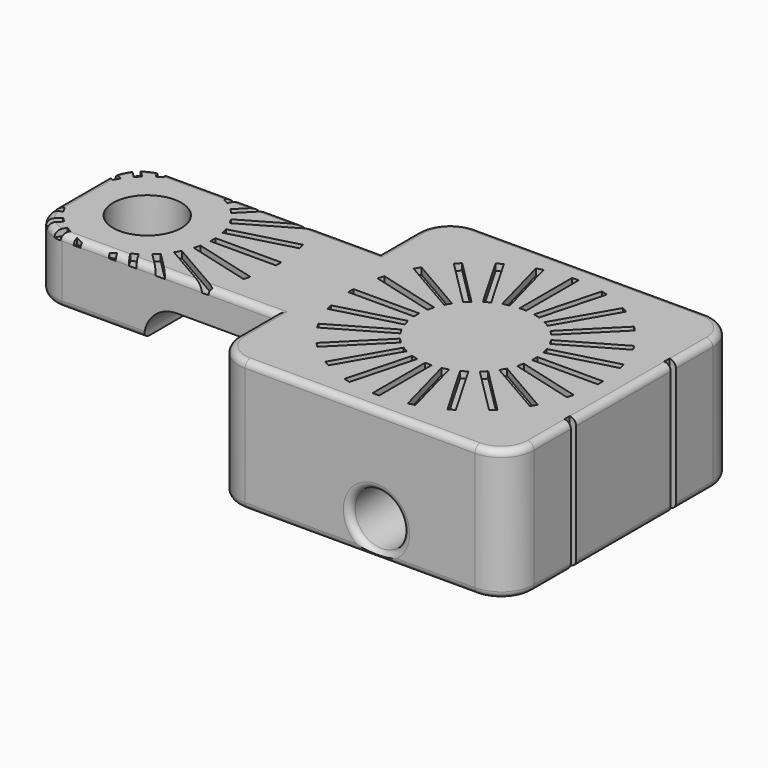
from build123d import *

# Parameters (mm, degrees)
F0_R         = 5.2
F1_DEPTH     = 20
F2_W         = 37.5
F2_H         = 20
F3_DEPTH     = 10
F4_R         = 4.05
F5_DEPTH     = 10
F6_R         = 4.05
F7_DEPTH     = 10
F8_T1_DEPTH  = 35
F8_T3_DEPTH  = 34
F8_T5_DEPTH  = 10
F8_T7_DEPTH  = 32.5
F8_T9_DEPTH  = 7
F8_T11_DEPTH = 7
F8_T14_ANGLE = 90
F8_T16_ANGLE = 90
F8_T18_ANGLE = 90
F8_T20_ANGLE = 90
F8_T26_ANGLE = 90
F8_T28_ANGLE = 90
F8_T30_ANGLE = 90
F8_T32_ANGLE = 90
F8_T34_ANGLE = 90
F8_T36_ANGLE = 90
F8_T38_ANGLE = 90
F8_T40_ANGLE = 90
F8_T45_DEPTH = 35
F8_T49_DEPTH = 9.5
F8_T56_DEPTH = 9.5
F8_T60_DEPTH = 35
F10_DEPTH    = 1
F11_W        = 20
F11_H        = 5
F12_DEPTH    = 32.0010001
F13_R        = 4.99999
F14_W        = 10
F14_H        = 1
F14_W_2      = 1
F14_H_2      = 10
F15_DEPTH    = 1
F16_W        = 2
F16_H        = 1
F17_DEPTH    = 20.0010001


# Not quite as in the source:
# - a fillet or chamfer that OpenCascade refuses, or shapes differently, is made with other operations: its cross-section is extruded or revolved along the edge and cut away or added
# - a fillet or chamfer is up to 0.001 mm smaller than in the source, because OpenCascade refuses the exact size


with BuildPart() as f1:
    # F0 (on Top) → F1 (new body)
    with BuildSketch(Plane.XY):
        with BuildLine():
            Line((-17.5, -22), (17.5, -22))
            ThreePointArc((17.5, -22), (21.0355339059, -20.5355339059), (22.5, -17))
            Line((22.5, -17), (22.5, 17))
            ThreePointArc((22.5, 17), (21.0355339059, 20.5355339059), (17.5, 22))
            Line((17.5, 22), (-17.5, 22))
            ThreePointArc((-17.5, 22), (-21.0355339059, 20.5355339059), (-22.5, 17))
            Line((-22.5, 17), (-22.5, 10))
            Line((-22.5, 10), (-55, 10))
            ThreePointArc((-55, 10), (-58.5355339059, 8.5355339059), (-60, 5))
            Line((-60, 5), (-60, -5))
            ThreePointArc((-60, -5), (-58.5355339059, -8.5355339059), (-55, -10))
            Line((-55, -10), (-22.5, -10))
            Line((-22.5, -10), (-22.5, -17))
            ThreePointArc((-22.5, -17), (-21.0355339059, -20.5355339059), (-17.5, -22))
        make_face()
        with Locations((-50, 0)):
            Circle(F0_R, mode=Mode.SUBTRACT)
    extrude(amount=F1_DEPTH)

    # F2 (on face) → F3 (cut)
    with BuildSketch(Plane(origin=(0, 0, 0), x_dir=(1, 0, 0), z_dir=(0, 0, -1))):
        with Locations((-41.25, 0)):
            Rectangle(F2_W, F2_H)
    extrude(amount=-F3_DEPTH, mode=Mode.SUBTRACT)

    # F4 (on face) → F5 (cut)
    with BuildSketch(Plane.XZ.offset(22)):
        with Locations((2.5, 5)):
            Circle(F4_R)
    extrude(amount=-F5_DEPTH, mode=Mode.SUBTRACT)

    # F6 (on face) → F7 (cut)
    with BuildSketch(Plane(origin=(0, 22, 0), x_dir=(-1, 0, 0), z_dir=(0, 1, 0))):
        with Locations((-2.5, 5)):
            Circle(F6_R)
    extrude(amount=-F7_DEPTH, mode=Mode.SUBTRACT)

    # F8: fillet of radius 1 on 18 edges, made by hand

    # F8_s2 → F8_t1 (cut)
    with BuildSketch(Plane.YZ.offset(-17.5)):
        with BuildLine():
            ThreePointArc((-22, 1), (-21.7071067812, 0.2928932188), (-21, 0))
            Line((-21, 0), (-22, 0))
            Line((-22, 0), (-22, 1))
        make_face()
        with BuildLine():
            ThreePointArc((21, 0), (21.7071067812, 0.2928932188), (22, 1))
            Line((22, 1), (22, 0))
            Line((22, 0), (21, 0))
        make_face()
        with BuildLine():
            ThreePointArc((21, 20), (21.7071067812, 19.7071067812), (22, 19))
            Line((22, 19), (22, 20))
            Line((22, 20), (21, 20))
        make_face()
        with BuildLine():
            ThreePointArc((-22, 19), (-21.7071067812, 19.7071067812), (-21, 20))
            Line((-21, 20), (-22, 20))
            Line((-22, 20), (-22, 19))
        make_face()
    extrude(amount=F8_T1_DEPTH, mode=Mode.SUBTRACT)

    # F8_s4 → F8_t3 (cut)
    with BuildSketch(Plane.XZ.offset(-17)):
        with BuildLine():
            ThreePointArc((21.5, 0), (22.2071067812, 0.2928932188), (22.5, 1))
            Line((22.5, 1), (22.5, 0))
            Line((22.5, 0), (21.5, 0))
        make_face()
        with BuildLine():
            ThreePointArc((-21.5, 0), (-22.2071067812, 0.2928932188), (-22.5, 1))
            Line((-22.5, 1), (-22.5, 0))
            Line((-22.5, 0), (-21.5, 0))
        make_face()
        with BuildLine():
            ThreePointArc((21.5, 20), (22.2071067812, 19.7071067812), (22.5, 19))
            Line((22.5, 19), (22.5, 20))
            Line((22.5, 20), (21.5, 20))
        make_face()
    extrude(amount=F8_T3_DEPTH, mode=Mode.SUBTRACT)

    # F8_s6 → F8_t5 (cut)
    with BuildSketch(Plane.XZ.offset(-5)):
        with BuildLine():
            ThreePointArc((-60, 11), (-59.7071067812, 10.2928932188), (-59, 10))
            Line((-59, 10), (-60, 10))
            Line((-60, 10), (-60, 11))
        make_face()
        with BuildLine():
            ThreePointArc((-59, 20), (-59.7071067812, 19.7071067812), (-60, 19))
            Line((-60, 19), (-60, 20))
            Line((-60, 20), (-59, 20))
        make_face()
    extrude(amount=F8_T5_DEPTH, mode=Mode.SUBTRACT)

    # F8_s8 → F8_t7 (cut)
    with BuildSketch(Plane.YZ.offset(-55)):
        with BuildLine():
            ThreePointArc((-9, 20), (-9.7071067812, 19.7071067812), (-10, 19))
            Line((-10, 19), (-10, 20))
            Line((-10, 20), (-9, 20))
        make_face()
        with BuildLine():
            ThreePointArc((9, 20), (9.7071067812, 19.7071067812), (10, 19))
            Line((10, 19), (10, 20))
            Line((10, 20), (9, 20))
        make_face()
        with BuildLine():
            ThreePointArc((10, 11), (9.7071067812, 10.2928932188), (9, 10))
            Line((9, 10), (10, 10))
            Line((10, 10), (10, 11))
        make_face()
        with BuildLine():
            ThreePointArc((-10, 11), (-9.7071067812, 10.2928932188), (-9, 10))
            Line((-9, 10), (-10, 10))
            Line((-10, 10), (-10, 11))
        make_face()
    extrude(amount=F8_T7_DEPTH, mode=Mode.SUBTRACT)

    # F8_s10 → F8_t9 (cut)
    with BuildSketch(Plane.XZ.offset(10)):
        with BuildLine():
            ThreePointArc((-21.5, 20), (-22.2071067812, 19.7071067812), (-22.5, 19))
            Line((-22.5, 19), (-22.5, 20))
            Line((-22.5, 20), (-21.5, 20))
        make_face()
    extrude(amount=F8_T9_DEPTH, mode=Mode.SUBTRACT)

    # F8_s12 → F8_t11 (cut)
    with BuildSketch(Plane.XZ.offset(-17)):
        with BuildLine():
            ThreePointArc((-21.5, 20), (-22.2071067812, 19.7071067812), (-22.5, 19))
            Line((-22.5, 19), (-22.5, 20))
            Line((-22.5, 20), (-21.5, 20))
        make_face()
    extrude(amount=F8_T11_DEPTH, mode=Mode.SUBTRACT)

    # F8_s13 → F8_t14 (revolve, cut)
    with BuildSketch(Plane.XZ.offset(17)):
        with BuildLine():
            ThreePointArc((-22.5, 1), (-22.2071067812, 0.2928932188), (-21.5, 0))
            Line((-21.5, 0), (-22.5, 0))
            Line((-22.5, 0), (-22.5, 1))
        make_face()
    revolve(axis=Axis((-17.5, -17, 0), (0, 0, 1)), revolution_arc=F8_T14_ANGLE, mode=Mode.SUBTRACT)

    # F8_s15 → F8_t16 (revolve, cut)
    with BuildSketch(Plane.YZ.offset(17.5)):
        with BuildLine():
            ThreePointArc((-21, 0), (-21.7071067812, 0.2928932188), (-22, 1))
            Line((-22, 1), (-22, 0))
            Line((-22, 0), (-21, 0))
        make_face()
    revolve(axis=Axis((17.5, -17, 0), (0, 0, 1)), revolution_arc=F8_T16_ANGLE, mode=Mode.SUBTRACT)

    # F8_s17 → F8_t18 (revolve, cut)
    with BuildSketch(Plane.XZ.offset(-17)):
        with BuildLine():
            ThreePointArc((21.5, 0), (22.2071067812, 0.2928932188), (22.5, 1))
            Line((22.5, 1), (22.5, 0))
            Line((22.5, 0), (21.5, 0))
        make_face()
    revolve(axis=Axis((17.5, 17, 0), (0, 0, 1)), revolution_arc=F8_T18_ANGLE, mode=Mode.SUBTRACT)

    # F8_s19 → F8_t20 (revolve, cut)
    with BuildSketch(Plane.YZ.offset(-17.5)):
        with BuildLine():
            ThreePointArc((21, 0), (21.7071067812, 0.2928932188), (22, 1))
            Line((22, 1), (22, 0))
            Line((22, 0), (21, 0))
        make_face()
    revolve(axis=Axis((-17.5, 17, 0), (0, 0, 1)), revolution_arc=F8_T20_ANGLE, mode=Mode.SUBTRACT)

    # F8_s21 → F8_t22 (revolve, cut)
    with BuildSketch(Plane.XY.offset(5)):
        with BuildLine():
            ThreePointArc((7.55, -22), (6.8428932188, -21.7071067812), (6.55, -21))
            Line((6.55, -21), (6.55, -22))
            Line((6.55, -22), (7.55, -22))
        make_face()
    revolve(axis=Axis((2.5, -22, 5), (0, -1, 0)), mode=Mode.SUBTRACT)

    # F8_s23 → F8_t24 (revolve, cut)
    with BuildSketch(Plane.XY.offset(5)):
        with BuildLine():
            ThreePointArc((-2.55, 22), (-1.8428932188, 21.7071067812), (-1.55, 21))
            Line((-1.55, 21), (-1.55, 22))
            Line((-1.55, 22), (-2.55, 22))
        make_face()
    revolve(axis=Axis((2.5, 22, 5), (0, 1, 0)), mode=Mode.SUBTRACT)

    # F8_s25 → F8_t26 (revolve, cut)
    with BuildSketch(Plane.XZ.offset(17)):
        with BuildLine():
            ThreePointArc((-22.5, 19), (-22.2071067812, 19.7071067812), (-21.5, 20))
            Line((-21.5, 20), (-22.5, 20))
            Line((-22.5, 20), (-22.5, 19))
        make_face()
    revolve(axis=Axis((-17.5, -17, 20), (0, 0, 1)), revolution_arc=F8_T26_ANGLE, mode=Mode.SUBTRACT)

    # F8_s27 → F8_t28 (revolve, cut)
    with BuildSketch(Plane.YZ.offset(17.5)):
        with BuildLine():
            ThreePointArc((-21, 20), (-21.7071067812, 19.7071067812), (-22, 19))
            Line((-22, 19), (-22, 20))
            Line((-22, 20), (-21, 20))
        make_face()
    revolve(axis=Axis((17.5, -17, 20), (0, 0, 1)), revolution_arc=F8_T28_ANGLE, mode=Mode.SUBTRACT)

    # F8_s29 → F8_t30 (revolve, cut)
    with BuildSketch(Plane.XZ.offset(-17)):
        with BuildLine():
            ThreePointArc((21.5, 20), (22.2071067812, 19.7071067812), (22.5, 19))
            Line((22.5, 19), (22.5, 20))
            Line((22.5, 20), (21.5, 20))
        make_face()
    revolve(axis=Axis((17.5, 17, 20), (0, 0, 1)), revolution_arc=F8_T30_ANGLE, mode=Mode.SUBTRACT)

    # F8_s31 → F8_t32 (revolve, cut)
    with BuildSketch(Plane.YZ.offset(-17.5)):
        with BuildLine():
            ThreePointArc((21, 20), (21.7071067812, 19.7071067812), (22, 19))
            Line((22, 19), (22, 20))
            Line((22, 20), (21, 20))
        make_face()
    revolve(axis=Axis((-17.5, 17, 20), (0, 0, 1)), revolution_arc=F8_T32_ANGLE, mode=Mode.SUBTRACT)

    # F8_s33 → F8_t34 (revolve, cut)
    with BuildSketch(Plane.XZ.offset(5)):
        with BuildLine():
            ThreePointArc((-59, 20), (-59.7071067812, 19.7071067812), (-60, 19))
            Line((-60, 19), (-60, 20))
            Line((-60, 20), (-59, 20))
        make_face()
    revolve(axis=Axis((-55, -5, 20), (0, 0, 1)), revolution_arc=F8_T34_ANGLE, mode=Mode.SUBTRACT)

    # F8_s35 → F8_t36 (revolve, cut)
    with BuildSketch(Plane.YZ.offset(-55)):
        with BuildLine():
            ThreePointArc((9, 20), (9.7071067812, 19.7071067812), (10, 19))
            Line((10, 19), (10, 20))
            Line((10, 20), (9, 20))
        make_face()
    revolve(axis=Axis((-55, 5, 20), (0, 0, 1)), revolution_arc=F8_T36_ANGLE, mode=Mode.SUBTRACT)

    # F8_s37 → F8_t38 (revolve, cut)
    with BuildSketch(Plane.YZ.offset(-55)):
        with BuildLine():
            ThreePointArc((-10, 11), (-9.7071067812, 10.2928932188), (-9, 10))
            Line((-9, 10), (-10, 10))
            Line((-10, 10), (-10, 11))
        make_face()
    revolve(axis=Axis((-55, -5, 10), (0, 0, -1)), revolution_arc=F8_T38_ANGLE, mode=Mode.SUBTRACT)

    # F8_s39 → F8_t40 (revolve, cut)
    with BuildSketch(Plane.XZ.offset(-5)):
        with BuildLine():
            ThreePointArc((-60, 11), (-59.7071067812, 10.2928932188), (-59, 10))
            Line((-59, 10), (-60, 10))
            Line((-60, 10), (-60, 11))
        make_face()
    revolve(axis=Axis((-55, 5, 10), (0, 0, -1)), revolution_arc=F8_T40_ANGLE, mode=Mode.SUBTRACT)


with BuildPart() as f8_tool43:
    # F8_s44 → F8_t45 (new body)
    with BuildSketch(Plane.YZ.offset(-55)):
        with BuildLine():
            ThreePointArc((-9, 20), (-9.7071067812, 19.7071067812), (-10, 19))
            Line((-10, 19), (-10, 20))
            Line((-10, 20), (-9, 20))
        make_face()
    extrude(amount=F8_T45_DEPTH)

    split(bisect_by=Plane.YZ.offset(-22.5), keep=Keep.TOP)


with BuildPart() as f8_tool47:
    # F8_s48 → F8_t49 (new body)
    with BuildSketch(Plane.XZ.offset(7.5)):
        with BuildLine():
            ThreePointArc((-21.5, 20), (-22.2071067812, 19.7071067812), (-22.5, 19))
            Line((-22.5, 19), (-22.5, 20))
            Line((-22.5, 20), (-21.5, 20))
        make_face()
    extrude(amount=F8_T49_DEPTH)

    split(bisect_by=Plane.XZ.offset(10), keep=Keep.BOTTOM)


with BuildPart() as f8_tool43_1:
    add(f8_tool43.part)

    # F8_t51: intersect F8_tool47
    add(f8_tool47.part, mode=Mode.INTERSECT)


with BuildPart() as f1_1:
    add(f1.part)

    # F8_t41: cut F8_tool43
    add(f8_tool43_1.part, mode=Mode.SUBTRACT)


with BuildPart() as f8_tool54:
    # F8_s55 → F8_t56 (new body)
    with BuildSketch(Plane.XZ.offset(-17)):
        with BuildLine():
            ThreePointArc((-21.5, 20), (-22.2071067812, 19.7071067812), (-22.5, 19))
            Line((-22.5, 19), (-22.5, 20))
            Line((-22.5, 20), (-21.5, 20))
        make_face()
    extrude(amount=F8_T56_DEPTH)

    split(bisect_by=Plane.XZ.offset(-10), keep=Keep.TOP)


with BuildPart() as f8_tool58:
    # F8_s59 → F8_t60 (new body)
    with BuildSketch(Plane.YZ.offset(-20)):
        with BuildLine():
            ThreePointArc((9, 20), (9.7071067812, 19.7071067812), (10, 19))
            Line((10, 19), (10, 20))
            Line((10, 20), (9, 20))
        make_face()
    extrude(amount=-F8_T60_DEPTH)

    split(bisect_by=Plane.YZ.offset(-22.5), keep=Keep.TOP)


with BuildPart() as f8_tool54_1:
    add(f8_tool54.part)

    # F8_t62: intersect F8_tool58
    add(f8_tool58.part, mode=Mode.INTERSECT)


with BuildPart() as f1_2:
    add(f1_1.part)

    # F8_t52: cut F8_tool54
    add(f8_tool54_1.part, mode=Mode.SUBTRACT)

    # F9 (on face) → F10 (cut)
    with BuildSketch(Plane.XY.offset(20)):
        with BuildLine():
            Line((8.9934199132, -0.5), (18.9934199132, -0.5))
            ThreePointArc((18.9934199132, -0.5), (19, 0), (18.9934199132, 0.5))
            Line((18.9934199132, 0.5), (8.9934199132, 0.5))
            Line((8.9934199132, 0.5), (8.9934199132, -0.5))
        make_face()
        with BuildLine():
            Line((8.8163860834, 1.844705441), (18.4756443463, 4.432895892))
            ThreePointArc((18.4756443463, 4.432895892), (18.3525906995, 4.9175618569), (18.2168253012, 5.3988217183))
            Line((18.2168253012, 5.3988217183), (8.5575670383, 2.8106312673))
            Line((8.5575670383, 2.8106312673), (8.8163860834, 1.844705441))
        make_face()
        with BuildLine():
            Line((8.0385301118, 4.0636972547), (16.6987841496, 9.0636972547))
            ThreePointArc((16.6987841496, 9.0636972547), (16.4544826719, 9.5), (16.1987841496, 9.9297226585))
            Line((16.1987841496, 9.9297226585), (7.5385301118, 4.9297226585))
            Line((7.5385301118, 4.9297226585), (8.0385301118, 4.0636972547))
        make_face()
        with BuildLine():
            Line((6.7128615973, 6.0057548161), (13.7839294092, 13.076822628))
            ThreePointArc((13.7839294092, 13.076822628), (13.4350288425, 13.4350288425), (13.076822628, 13.7839294092))
            Line((13.076822628, 13.7839294092), (6.0057548161, 6.7128615973))
            Line((6.0057548161, 6.7128615973), (6.7128615973, 6.0057548161))
        make_face()
        with BuildLine():
            Line((4.9297226585, 7.5385301118), (9.9297226585, 16.1987841496))
            ThreePointArc((9.9297226585, 16.1987841496), (9.5, 16.4544826719), (9.0636972547, 16.6987841496))
            Line((9.0636972547, 16.6987841496), (4.0636972547, 8.0385301118))
            Line((4.0636972547, 8.0385301118), (4.9297226585, 7.5385301118))
        make_face()
        with BuildLine():
            Line((2.8106312673, 8.5575670383), (5.3988217183, 18.2168253012))
            ThreePointArc((5.3988217183, 18.2168253012), (4.9175618569, 18.3525906995), (4.432895892, 18.4756443463))
            Line((4.432895892, 18.4756443463), (1.844705441, 8.8163860834))
            Line((1.844705441, 8.8163860834), (2.8106312673, 8.5575670383))
        make_face()
        with BuildLine():
            Line((0.5, 8.9934199132), (0.5, 18.9934199132))
            ThreePointArc((0.5, 18.9934199132), (0, 19), (-0.5, 18.9934199132))
            Line((-0.5, 18.9934199132), (-0.5, 8.9934199132))
            Line((-0.5, 8.9934199132), (0.5, 8.9934199132))
        make_face()
        with BuildLine():
            Line((-1.844705441, 8.8163860834), (-4.432895892, 18.4756443463))
            ThreePointArc((-4.432895892, 18.4756443463), (-4.9175618569, 18.3525906995), (-5.3988217183, 18.2168253012))
            Line((-5.3988217183, 18.2168253012), (-2.8106312673, 8.5575670383))
            Line((-2.8106312673, 8.5575670383), (-1.844705441, 8.8163860834))
        make_face()
        with BuildLine():
            Line((-4.0636972547, 8.0385301118), (-9.0636972547, 16.6987841496))
            ThreePointArc((-9.0636972547, 16.6987841496), (-9.5, 16.4544826719), (-9.9297226585, 16.1987841496))
            Line((-9.9297226585, 16.1987841496), (-4.9297226585, 7.5385301118))
            Line((-4.9297226585, 7.5385301118), (-4.0636972547, 8.0385301118))
        make_face()
        with BuildLine():
            Line((-6.0057548161, 6.7128615973), (-13.076822628, 13.7839294092))
            ThreePointArc((-13.076822628, 13.7839294092), (-13.4350288425, 13.4350288425), (-13.7839294092, 13.076822628))
            Line((-13.7839294092, 13.076822628), (-6.7128615973, 6.0057548161))
            Line((-6.7128615973, 6.0057548161), (-6.0057548161, 6.7128615973))
        make_face()
        with BuildLine():
            Line((-7.5385301118, 4.9297226585), (-16.1987841496, 9.9297226585))
            ThreePointArc((-16.1987841496, 9.9297226585), (-16.4544826719, 9.5), (-16.6987841496, 9.0636972547))
            Line((-16.6987841496, 9.0636972547), (-8.0385301118, 4.0636972547))
            Line((-8.0385301118, 4.0636972547), (-7.5385301118, 4.9297226585))
        make_face()
        with BuildLine():
            Line((-8.5575670383, 2.8106312673), (-18.2168253012, 5.3988217183))
            ThreePointArc((-18.2168253012, 5.3988217183), (-18.3525906995, 4.9175618569), (-18.4756443463, 4.432895892))
            Line((-18.4756443463, 4.432895892), (-8.8163860834, 1.844705441))
            Line((-8.8163860834, 1.844705441), (-8.5575670383, 2.8106312673))
        make_face()
        with BuildLine():
            Line((-8.9934199132, 0.5), (-18.9934199132, 0.5))
            ThreePointArc((-18.9934199132, 0.5), (-19, 0), (-18.9934199132, -0.5))
            Line((-18.9934199132, -0.5), (-8.9934199132, -0.5))
            Line((-8.9934199132, -0.5), (-8.9934199132, 0.5))
        make_face()
        with BuildLine():
            Line((-8.8163860834, -1.844705441), (-18.4756443463, -4.432895892))
            ThreePointArc((-18.4756443463, -4.432895892), (-18.3525906995, -4.9175618569), (-18.2168253012, -5.3988217183))
            Line((-18.2168253012, -5.3988217183), (-8.5575670383, -2.8106312673))
            Line((-8.5575670383, -2.8106312673), (-8.8163860834, -1.844705441))
        make_face()
        with BuildLine():
            Line((-8.0385301118, -4.0636972547), (-16.6987841496, -9.0636972547))
            ThreePointArc((-16.6987841496, -9.0636972547), (-16.4544826719, -9.5), (-16.1987841496, -9.9297226585))
            Line((-16.1987841496, -9.9297226585), (-7.5385301118, -4.9297226585))
            Line((-7.5385301118, -4.9297226585), (-8.0385301118, -4.0636972547))
        make_face()
        with BuildLine():
            Line((-6.7128615973, -6.0057548161), (-13.7839294092, -13.076822628))
            ThreePointArc((-13.7839294092, -13.076822628), (-13.4350288425, -13.4350288425), (-13.076822628, -13.7839294092))
            Line((-13.076822628, -13.7839294092), (-6.0057548161, -6.7128615973))
            Line((-6.0057548161, -6.7128615973), (-6.7128615973, -6.0057548161))
        make_face()
        with BuildLine():
            Line((-4.9297226585, -7.5385301118), (-9.9297226585, -16.1987841496))
            ThreePointArc((-9.9297226585, -16.1987841496), (-9.5, -16.4544826719), (-9.0636972547, -16.6987841496))
            Line((-9.0636972547, -16.6987841496), (-4.0636972547, -8.0385301118))
            Line((-4.0636972547, -8.0385301118), (-4.9297226585, -7.5385301118))
        make_face()
        with BuildLine():
            Line((-2.8106312673, -8.5575670383), (-5.3988217183, -18.2168253012))
            ThreePointArc((-5.3988217183, -18.2168253012), (-4.9175618569, -18.3525906995), (-4.432895892, -18.4756443463))
            Line((-4.432895892, -18.4756443463), (-1.844705441, -8.8163860834))
            Line((-1.844705441, -8.8163860834), (-2.8106312673, -8.5575670383))
        make_face()
        with BuildLine():
            Line((-0.5, -8.9934199132), (-0.5, -18.9934199132))
            ThreePointArc((-0.5, -18.9934199132), (0, -19), (0.5, -18.9934199132))
            Line((0.5, -18.9934199132), (0.5, -8.9934199132))
            Line((0.5, -8.9934199132), (-0.5, -8.9934199132))
        make_face()
        with BuildLine():
            Line((1.844705441, -8.8163860834), (4.432895892, -18.4756443463))
            ThreePointArc((4.432895892, -18.4756443463), (4.9175618569, -18.3525906995), (5.3988217183, -18.2168253012))
            Line((5.3988217183, -18.2168253012), (2.8106312673, -8.5575670383))
            Line((2.8106312673, -8.5575670383), (1.844705441, -8.8163860834))
        make_face()
        with BuildLine():
            Line((4.0636972547, -8.0385301118), (9.0636972547, -16.6987841496))
            ThreePointArc((9.0636972547, -16.6987841496), (9.5, -16.4544826719), (9.9297226585, -16.1987841496))
            Line((9.9297226585, -16.1987841496), (4.9297226585, -7.5385301118))
            Line((4.9297226585, -7.5385301118), (4.0636972547, -8.0385301118))
        make_face()
        with BuildLine():
            Line((6.0057548161, -6.7128615973), (13.076822628, -13.7839294092))
            ThreePointArc((13.076822628, -13.7839294092), (13.4350288425, -13.4350288425), (13.7839294092, -13.076822628))
            Line((13.7839294092, -13.076822628), (6.7128615973, -6.0057548161))
            Line((6.7128615973, -6.0057548161), (6.0057548161, -6.7128615973))
        make_face()
        with BuildLine():
            Line((7.5385301118, -4.9297226585), (16.1987841496, -9.9297226585))
            ThreePointArc((16.1987841496, -9.9297226585), (16.4544826719, -9.5), (16.6987841496, -9.0636972547))
            Line((16.6987841496, -9.0636972547), (8.0385301118, -4.0636972547))
            Line((8.0385301118, -4.0636972547), (7.5385301118, -4.9297226585))
        make_face()
        with BuildLine():
            Line((8.5575670383, -2.8106312673), (18.2168253012, -5.3988217183))
            ThreePointArc((18.2168253012, -5.3988217183), (18.3525906995, -4.9175618569), (18.4756443463, -4.432895892))
            Line((18.4756443463, -4.432895892), (8.8163860834, -1.844705441))
            Line((8.8163860834, -1.844705441), (8.5575670383, -2.8106312673))
        make_face()
    extrude(amount=-F10_DEPTH, mode=Mode.SUBTRACT)

    # F11 (on face) → F12 (cut, through all)
    with BuildSketch(Plane.XZ.offset(10)):
        with Locations((-32.5, 12.5)):
            Rectangle(F11_W, F11_H)
    extrude(amount=-F12_DEPTH, mode=Mode.SUBTRACT)

    # F13 (radius 5 in the source; OpenCascade refuses exactly that, so slightly less here)
    f13_edges = [f1_2.edges().sort_by_distance(p)[0] for p in [
        (-42.5, 0, 15),
        (-22.5, 0, 15),
    ]]
    fillet(f13_edges, radius=F13_R)

    # F14 (on face) → F15 (cut)
    with BuildSketch(Plane.XY.offset(20)):
        with Locations((-35, 0)):
            Rectangle(F14_W, F14_H)
        Polygon((-30.8108929968, 5.6593438152), (-40.4701512597, 3.0711533642), (-40.2113322146, 2.1052275379), (-30.5520739517, 4.6934179889), align=None)
        Polygon((-32.9294919243, 10.4330127019), (-41.5897459622, 5.4330127019), (-41.0897459622, 4.5669872981), (-32.4294919243, 9.5669872981), align=None)
        Polygon((-36.2114177669, 14.4956890143), (-43.2824855787, 7.4246212025), (-42.5753787975, 6.7175144213), (-35.5043109857, 13.7885822331), align=None)
        Polygon((-40.4330127019, 17.5705080757), (-45.4330127019, 8.9102540378), (-44.5669872981, 8.4102540378), (-39.5669872981, 17.0705080757), align=None)
        Polygon((-45.3065820111, 19.4479260483), (-47.8947724621, 9.7886677854), (-46.9288466358, 9.5298487403), (-44.3406561848, 19.1891070032), align=None)
        with Locations((-50, 15)):
            Rectangle(F14_W_2, F14_H_2)
        Polygon((-55.6593438152, 19.1891070032), (-53.0711533642, 9.5298487403), (-52.1052275379, 9.7886677854), (-54.6934179889, 19.4479260483), align=None)
        Polygon((-60.4330127019, 17.0705080757), (-55.4330127019, 8.4102540378), (-54.5669872981, 8.9102540378), (-59.5669872981, 17.5705080757), align=None)
        Polygon((-64.4956890143, 13.7885822331), (-57.4246212025, 6.7175144213), (-56.7175144213, 7.4246212025), (-63.7885822331, 14.4956890143), align=None)
        Polygon((-67.5705080757, 9.5669872981), (-58.9102540378, 4.5669872981), (-58.4102540378, 5.4330127019), (-67.0705080757, 10.4330127019), align=None)
        Polygon((-69.4479260483, 4.6934179889), (-59.7886677854, 2.1052275379), (-59.5298487403, 3.0711533642), (-69.1891070032, 5.6593438152), align=None)
        with Locations((-65, 0)):
            Rectangle(F14_W, F14_H)
        Polygon((-69.1891070032, -5.6593438152), (-59.5298487403, -3.0711533642), (-59.7886677854, -2.1052275379), (-69.4479260483, -4.6934179889), align=None)
        Polygon((-67.0705080757, -10.4330127019), (-58.4102540378, -5.4330127019), (-58.9102540378, -4.5669872981), (-67.5705080757, -9.5669872981), align=None)
        Polygon((-63.7885822331, -14.4956890143), (-56.7175144213, -7.4246212025), (-57.4246212025, -6.7175144213), (-64.4956890143, -13.7885822331), align=None)
        Polygon((-59.5669872981, -17.5705080757), (-54.5669872981, -8.9102540378), (-55.4330127019, -8.4102540378), (-60.4330127019, -17.0705080757), align=None)
        Polygon((-54.6934179889, -19.4479260483), (-52.1052275379, -9.7886677854), (-53.0711533642, -9.5298487403), (-55.6593438152, -19.1891070032), align=None)
        with Locations((-50, -15)):
            Rectangle(F14_W_2, F14_H_2)
        Polygon((-44.3406561848, -19.1891070032), (-46.9288466358, -9.5298487403), (-47.8947724621, -9.7886677854), (-45.3065820111, -19.4479260483), align=None)
        Polygon((-39.5669872981, -17.0705080757), (-44.5669872981, -8.4102540378), (-45.4330127019, -8.9102540378), (-40.4330127019, -17.5705080757), align=None)
        Polygon((-35.5043109857, -13.7885822331), (-42.5753787975, -6.7175144213), (-43.2824855787, -7.4246212025), (-36.2114177669, -14.4956890143), align=None)
        Polygon((-32.4294919243, -9.5669872981), (-41.0897459622, -4.5669872981), (-41.5897459622, -5.4330127019), (-32.9294919243, -10.4330127019), align=None)
        Polygon((-30.5520739517, -4.6934179889), (-40.2113322146, -2.1052275379), (-40.4701512597, -3.0711533642), (-30.8108929968, -5.6593438152), align=None)
    extrude(amount=-F15_DEPTH, mode=Mode.SUBTRACT)

    # F16 (on face) → F17 (cut, through all)
    with BuildSketch(Plane.XY.offset(20)):
        with Locations((22.5, 9.5)):
            Rectangle(F16_W, F16_H)
        with Locations((22.5, -9.5)):
            Rectangle(F16_W, F16_H)
    extrude(amount=-F17_DEPTH, mode=Mode.SUBTRACT)


solid = f1_2.part
